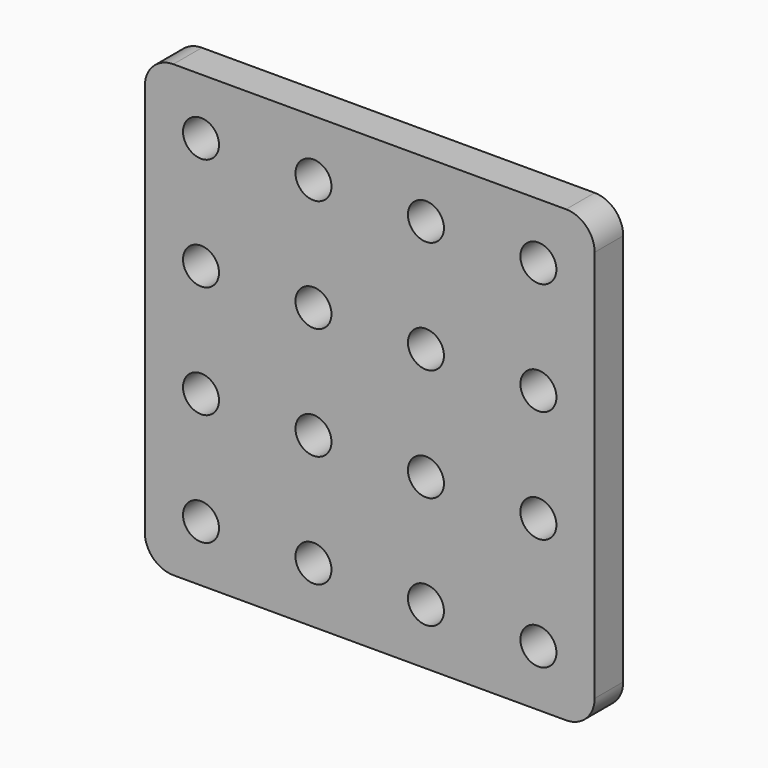
from build123d import *

# Parameters (mm, degrees)
F0_R     = 1.6
F1_DEPTH = 3.175


# Not quite as in the source:
# - a length typed as a fraction of an inch, garbled in the dataset ("3 / 203.2 mm" for 3/8 in), is restored


with BuildPart() as f1:
    # F0 (on Front) → F1 (new body)
    with BuildSketch(Plane.XZ):
        with BuildLine():
            Line((37.46, 0), (2.54, 0))
            ThreePointArc((2.54, 0), (0.7439487758, -0.7439487758), (0, -2.54))
            Line((0, -2.54), (0, -37.46))
            ThreePointArc((0, -37.46), (0.7439487758, -39.2560512242), (2.54, -40))
            Line((2.54, -40), (37.46, -40))
            ThreePointArc((37.46, -40), (39.2560512242, -39.2560512242), (40, -37.46))
            Line((40, -37.46), (40, -2.54))
            ThreePointArc((40, -2.54), (39.2560512242, -0.7439487758), (37.46, 0))
        make_face()
        with Locations((5, -35)):
            Circle(F0_R, mode=Mode.SUBTRACT)
        with Locations((15, -35)):
            Circle(F0_R, mode=Mode.SUBTRACT)
        with Locations((5, -25)):
            Circle(F0_R, mode=Mode.SUBTRACT)
        with Locations((15, -25)):
            Circle(F0_R, mode=Mode.SUBTRACT)
        with Locations((25, -35)):
            Circle(F0_R, mode=Mode.SUBTRACT)
        with Locations((35, -35)):
            Circle(F0_R, mode=Mode.SUBTRACT)
        with Locations((25, -25)):
            Circle(F0_R, mode=Mode.SUBTRACT)
        with Locations((35, -25)):
            Circle(F0_R, mode=Mode.SUBTRACT)
        with Locations((5, -15)):
            Circle(F0_R, mode=Mode.SUBTRACT)
        with Locations((15, -15)):
            Circle(F0_R, mode=Mode.SUBTRACT)
        with Locations((5, -5)):
            Circle(F0_R, mode=Mode.SUBTRACT)
        with Locations((15, -5)):
            Circle(F0_R, mode=Mode.SUBTRACT)
        with Locations((25, -15)):
            Circle(F0_R, mode=Mode.SUBTRACT)
        with Locations((35, -15)):
            Circle(F0_R, mode=Mode.SUBTRACT)
        with Locations((25, -5)):
            Circle(F0_R, mode=Mode.SUBTRACT)
        with Locations((35, -5)):
            Circle(F0_R, mode=Mode.SUBTRACT)
    extrude(amount=F1_DEPTH)


solid = f1.part
